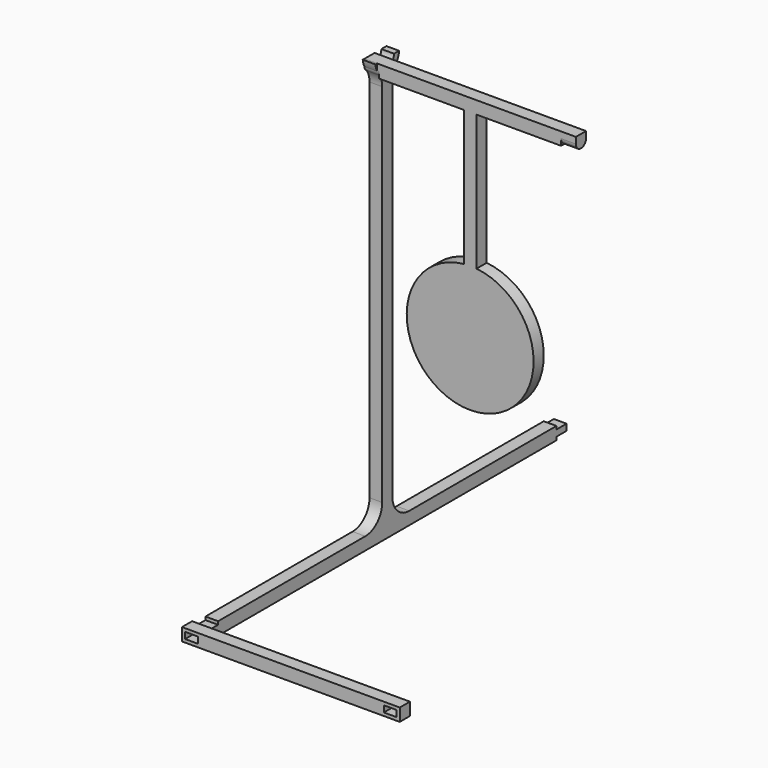
from build123d import *

# Parameters (mm, degrees)
F1_DEPTH    = 3
F2_T1_DEPTH = 3
F2_T3_DEPTH = 3
F2_T5_DEPTH = 13.0928039389
F2_T7_DEPTH = 13.0928039389
F3_R        = 5
F4_W        = 3
F4_H        = 1.5
F5_DEPTH    = 3
F7_DEPTH    = 3
F9_DEPTH    = 3.5


# Not quite as in the source:
# - a fillet or chamfer that OpenCascade refuses, or shapes differently, is made with other operations: its cross-section is extruded or revolved along the edge and cut away or added


with BuildPart() as f1:
    # F0 (on Right) → F1 (new body)
    with BuildSketch(Plane.YZ):
        with BuildLine():
            ThreePointArc((0, 98), (-1.4142135624, 98.5857864376), (-2, 100))
            Line((-2, 100), (-3.5, 100))
            Line((-3.5, 100), (-3.5, 98.5))
            Line((-3.5, 98.5), (-1.5, 96.5))
            Line((-1.5, 96.5), (-1.5, 3))
            Line((-1.5, 3), (-50, 3))
            Line((-50, 3), (-50, 2.25))
            Line((-50, 2.25), (-53, 2.25))
            Line((-53, 2.25), (-53, 0.75))
            Line((-53, 0.75), (-50, 0.75))
            Line((-50, 0.75), (-50, 0))
            Line((-50, 0), (0, 0))
            Line((0, 0), (50, 0))
            Line((50, 0), (50, 0.75))
            Line((50, 0.75), (53, 0.75))
            Line((53, 0.75), (53, 2.25))
            Line((53, 2.25), (50, 2.25))
            Line((50, 2.25), (50, 3))
            Line((50, 3), (1.5, 3))
            Line((1.5, 3), (1.5, 96.5))
            Line((1.5, 96.5), (3.5, 98.5))
            Line((3.5, 98.5), (3.5, 100))
            Line((3.5, 100), (2, 100))
            ThreePointArc((2, 100), (1.4142135624, 98.5857864376), (0, 98))
        make_face()
    extrude(amount=F1_DEPTH)

    # F2: fillet of radius 5 on 4 edges, made by hand

    # F2_s2 → F2_t1 (join)
    with BuildSketch(Plane.YZ):
        with BuildLine():
            ThreePointArc((1.5, 8), (2.9644660941, 4.4644660941), (6.5, 3))
            Line((6.5, 3), (1.5, 3))
            Line((1.5, 3), (1.5, 8))
        make_face()
    extrude(amount=F2_T1_DEPTH)

    # F2_s4 → F2_t3 (join)
    with BuildSketch(Plane.YZ):
        with BuildLine():
            ThreePointArc((-1.5, 8), (-2.9644660941, 4.4644660941), (-6.5, 3))
            Line((-6.5, 3), (-1.5, 3))
            Line((-1.5, 3), (-1.5, 8))
        make_face()
    extrude(amount=F2_T3_DEPTH)

    # F2_s6 → F2_t5 (cut)
    with BuildSketch(Plane.YZ.offset(-5.0464019695)):
        with BuildLine():
            ThreePointArc((3.5, 100), (3.0313524106, 98.4168612226), (2.0726619787, 97.0726619787))
            Line((2.0726619787, 97.0726619787), (3.5, 98.5))
            Line((3.5, 98.5), (3.5, 100))
        make_face()
    extrude(amount=F2_T5_DEPTH, mode=Mode.SUBTRACT)

    # F2_s8 → F2_t7 (cut)
    with BuildSketch(Plane.YZ.offset(-5.0464019695)):
        with BuildLine():
            ThreePointArc((-2.0726619787, 97.0726619787), (-3.0313524106, 98.4168612226), (-3.5, 100))
            Line((-3.5, 100), (-3.5, 98.5))
            Line((-3.5, 98.5), (-2.0726619787, 97.0726619787))
        make_face()
    extrude(amount=F2_T7_DEPTH, mode=Mode.SUBTRACT)

    # F3
    f3_edges = [f1.edges().sort_by_distance(p)[0] for p in [
        (1.5, -1.5, 96.5),
        (1.5, 1.5, 96.5),
    ]]
    fillet(f3_edges, radius=F3_R)


with BuildPart() as f5:
    # F4 (on face) → F5 (new body)
    with BuildSketch(Plane.XZ.offset(53)):
        Polygon((-0.75, 0), (0, 0), (25, 0), (50, 0), (50.75, 0), (50.75, 3), (50, 3), (47, 3), (25, 3), (3, 3), (0, 3), (-0.75, 3), align=None)
        with Locations((1.5, 1.5)):
            Rectangle(F4_W, F4_H, mode=Mode.SUBTRACT)
        with Locations((48.5, 1.5)):
            Rectangle(F4_W, F4_H, mode=Mode.SUBTRACT)
    extrude(amount=F5_DEPTH)


with BuildPart() as f7:
    # F6 (on Front) → F7 (new body)
    with BuildSketch(Plane.XZ):
        with BuildLine():
            Line((25, 64.9248115566), (25, 100))
            Line((25, 100), (0, 100))
            Line((0, 100), (0, 97))
            Line((0, 97), (23.5, 97))
            Line((23.5, 97), (23.5, 64.9248115566))
            ThreePointArc((23.5, 64.9248115566), (10.0188089033, 49.2490583741), (25, 35))
            Line((25, 35), (25, 64.9248115566))
        make_face()
    extrude(amount=F7_DEPTH)

    # F8 (on face) → F9 (cut)
    with BuildSketch(Plane(origin=(0, 0, 0), x_dir=(0, -1, 0), z_dir=(-1, 0, 0))):
        with BuildLine():
            Line((3, 97), (3, 98.5))
            ThreePointArc((3, 98.5), (2.5606601718, 97.4393398282), (1.5, 97))
            Line((1.5, 97), (3, 97))
        make_face()
        with BuildLine():
            Line((0, 97), (1.5, 97))
            ThreePointArc((1.5, 97), (0.4393398282, 97.4393398282), (0, 98.5))
            Line((0, 98.5), (0, 97))
        make_face()
    extrude(amount=-F9_DEPTH, mode=Mode.SUBTRACT)

    # F10: F7 across face


with BuildPart() as f7_1:
    add(f7.part)
    add(f7.part.mirror(Plane(origin=(25, -1.5, 67.5), x_dir=(0, 1, 0), z_dir=(1, 0, 0))))


solid = Compound([f1.part, f5.part, f7_1.part])
